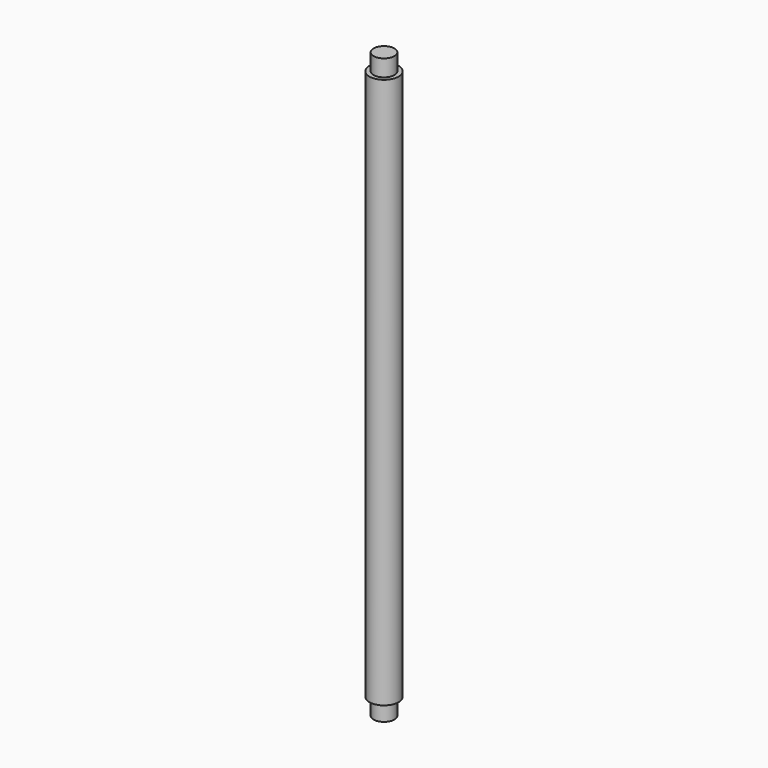
from build123d import *

# Parameters (mm, degrees)
F0_R     = 3.5
F1_DEPTH = 70
F2_R     = 3.5
F2_R_2   = 2.5
F3_DEPTH = 4


# Not quite as in the source:
# - a pattern or mirror of a feature is missing from the dataset's text; its kind, count and spacing are read off the source's solid


with BuildPart() as f1:
    # F0 (on Top) → F1 (new body, symmetric)
    with BuildSketch(Plane.XY):
        Circle(F0_R)
    extrude(amount=F1_DEPTH, both=True)

    # F2 (on face) → F3 (cut)
    with BuildSketch(Plane.XY.offset(70)):
        Circle(F2_R)
        Circle(F2_R_2, mode=Mode.SUBTRACT)
    f3 = extrude(amount=-F3_DEPTH, mode=Mode.SUBTRACT)

    # F3_copies: F3 across plane
    add(f3.mirror(Plane(origin=(0, 0, 0), x_dir=(-1, 0, 0), z_dir=(0, 0, -1))), mode=Mode.SUBTRACT)


solid = f1.part
